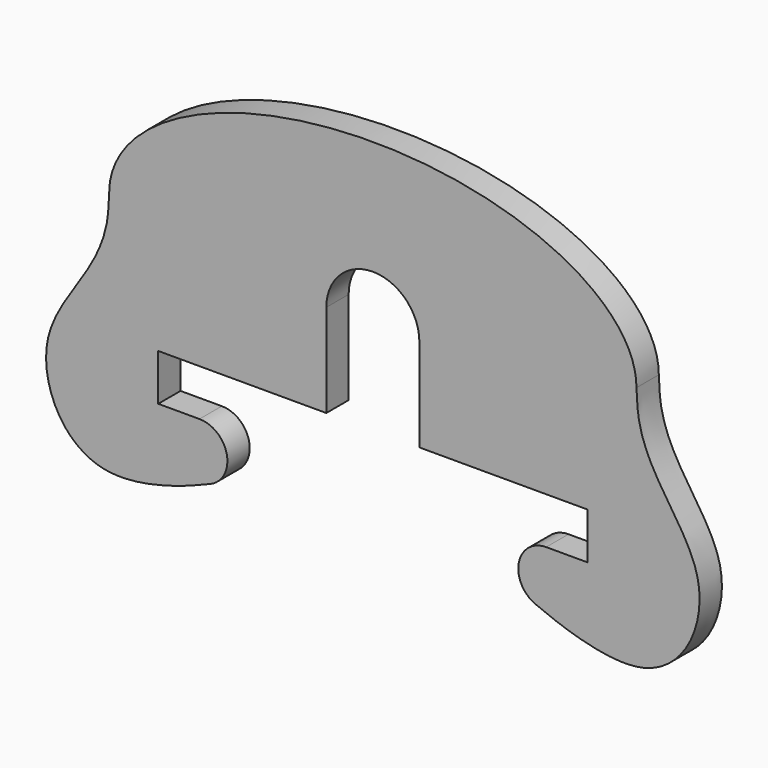
from build123d import *

# Parameters (mm, degrees)
F1_DEPTH = 3


# Not quite as in the source:
# - ends of sketch curves that miss each other by under 0.0002 mm in the source are joined
# - the dataset's text gives a spline's control points without its knots; the knots are read off the source's solid


with BuildPart() as f1:
    # F0 (on Front) → F1 (new body)
    with BuildSketch(Plane.XZ):
        with BuildLine():
            Line((-18.631138, -12.039077), (-23.065, -12.039077))
            Line((-23.065, -12.039077), (-23.065, -7.039077))
            Line((-23.065, -7.039077), (-5, -7.039077))
            Line((-5, -7.039077), (-5, 2.960923))
            ThreePointArc((-5, 2.960923), (0, 7.960923), (5, 2.960923))
            Line((5, 2.960923), (5, -7.039077))
            Line((5, -7.039077), (23.065, -7.039077))
            Line((23.065, -7.039077), (23.065, -12.039077))
            Line((23.065, -12.039077), (18.631137, -12.039077))
            ThreePointArc((18.631137, -12.039077), (15.6930952866, -14.4325204153), (17.4430779685, -17.7938030731))
            add(Edge.make_bspline(
                [(28.334969, 6.202538), (28.382769, 5.719314), (28.407006, -1.378841), (38.47544, -8.061034), (31.583633, -23.110185), (20.19345, -18.979985), (17.4430779685, -17.7938030731)],
                knots=[26.688985, 26.688985, 26.688985, 26.688985, 28.557776, 42.872008, 54.1154, 62.665306, 62.665306, 62.665306, 62.665306], degree=3))
            add(Edge.make_bspline(
                [(28.334969, 6.202538), (28.334969, 20.2509254333), (-4.9078e-06, 20.250923), (-28.3349788155, 20.2509205667), (-28.334969, 6.2025331335)],
                knots=[0, 0, 0, 1.5707965, 1.5707965, 3.141593, 3.141593, 3.141593], degree=2, weights=[1, 0.7071067199, 1, 0.7071067199, 1]))
            add(Edge.make_bspline(
                [(-28.334969, 6.2025331335), (-28.382769, 5.719314), (-28.407006, -1.378841), (-38.47544, -8.061034), (-31.583633, -23.110185), (-20.193451, -18.979985), (-17.443078, -17.793803)],
                knots=[26.688985, 26.688985, 26.688985, 26.688985, 28.557776, 42.872008, 54.1154, 62.665306, 62.665306, 62.665306, 62.665306], degree=3))
            ThreePointArc((-17.443078, -17.793803), (-15.6930963794, -14.4325199657), (-18.631138, -12.039077))
        make_face()
    extrude(amount=F1_DEPTH)


solid = f1.part
